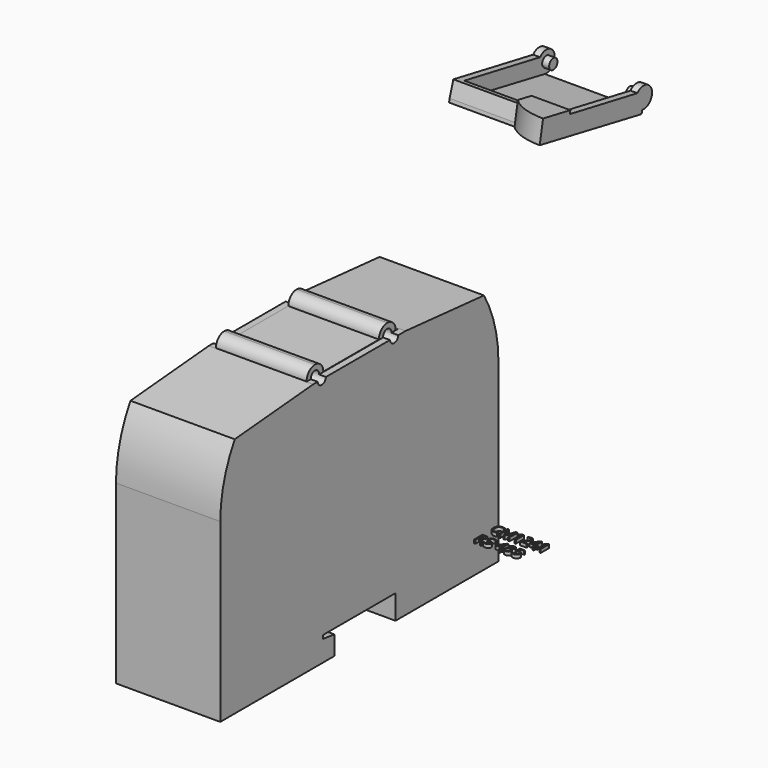
from build123d import *

# Parameters (mm, degrees)
F0_W          = 100
F0_H          = 75
F1_DEPTH      = 15
F3_DEPTH      = 34.2
F5_DEPTH      = 38.1
F6_W          = 4
F6_H          = 12
F7_DEPTH      = 10
F9_DEPTH      = 30
F10_W         = 26
F10_H         = 30.2941333291
F10_H_2       = 4.7058666709
F11_DEPTH     = 25
F12_R         = 1.5
F13_DEPTH     = 2
F14_R         = 1.5
F15_DEPTH     = 2
F16_W         = 26
F16_H         = 30.2941333291
F17_DEPTH     = 1
F19_DEPTH     = 6.4
F20_TEXT_SIZE = 4.1666666667
F21_DEPTH     = 1
F23_DEPTH     = 97.5
F25_DEPTH     = 45


# Not quite as in the source:
# - a feature names something its author has since deleted; it is built from what else it names
# - Text() gives the source's letters only with a copy of the font that has no kerning and outlines rounded to 1/6400 em; it was checked with that copy


with BuildPart() as f1:
    # F0 (on Right) → F1 (new body, symmetric)
    with BuildSketch(Plane.YZ):
        Rectangle(F0_W, F0_H)
    extrude(amount=F1_DEPTH, both=True)

    # F2 (on face) → F3 (cut)
    with BuildSketch(Plane.YZ.offset(15)):
        with BuildLine():
            ThreePointArc((-16.5, 34.5), (-15.62132033, 36.6213203571), (-13.4999999617, 37.5))
            Line((-13.4999999617, 37.5), (-50, 37.5))
            Line((-50, 37.5), (-50, 31.5))
            Line((-50, 31.5), (-16.4987426642, 34.4131528118))
            ThreePointArc((-16.4987426642, 34.4131528118), (-16.4996856496, 34.4565718554), (-16.5, 34.5))
        make_face()
        with BuildLine():
            ThreePointArc((12.5000000383, 37.5), (14.6213203571, 36.62132033), (15.5, 34.5))
            Line((15.5, 34.5), (50, 31.5))
            Line((50, 31.5), (50, 37.5))
            Line((50, 37.5), (12.5000000383, 37.5))
        make_face()
        with BuildLine():
            Line((-10.5, 34.5), (9.5, 34.5))
            ThreePointArc((9.5, 34.5), (10.37867967, 36.6213203571), (12.5000000383, 37.5))
            Line((12.5000000383, 37.5), (-13.4999999617, 37.5))
            ThreePointArc((-13.4999999617, 37.5), (-11.3786796429, 36.62132033), (-10.5, 34.5))
        make_face()
        with BuildLine():
            ThreePointArc((-15, 34.5), (-13.5, 33), (-12, 34.5))
            Line((-12, 34.5), (-15, 34.5))
        make_face()
        with BuildLine():
            Line((-15, 34.5), (-12, 34.5))
            ThreePointArc((-12, 34.5), (-13.5, 36), (-15, 34.5))
        make_face()
        with BuildLine():
            Line((14, 34.5), (11, 34.5))
            ThreePointArc((11, 34.5), (12.5, 33), (14, 34.5))
        make_face()
        with BuildLine():
            ThreePointArc((14, 34.5), (12.5, 36), (11, 34.5))
            Line((11, 34.5), (14, 34.5))
        make_face()
    extrude(amount=-F3_DEPTH, mode=Mode.SUBTRACT)

    # F4 (on face) → F5 (cut)
    with BuildSketch(Plane.YZ.offset(15)):
        with BuildLine():
            ThreePointArc((44.7955449747, 31.9525613065), (48.6477397083, 22.9432016728), (50, 13.2385967153))
            Line((50, 13.2385967153), (50, 31.5))
            Line((50, 31.5), (44.7955449747, 31.9525613065))
        make_face()
        with BuildLine():
            Line((-50, 31.5), (-50, 13.2385967153))
            ThreePointArc((-50, 13.2385967153), (-48.6477397083, 22.9432016728), (-44.7955449747, 31.9525613065))
            Line((-44.7955449747, 31.9525613065), (-50, 31.5))
        make_face()
    extrude(amount=-F5_DEPTH, mode=Mode.SUBTRACT)

    # F6 (on face) → F7 (cut)
    with BuildSketch(Plane(origin=(0, 50, 0), x_dir=(-1, 0, 0), z_dir=(0, 1, 0))):
        with Locations((-8, 2.2385967153)):
            Rectangle(F6_W, F6_H)
        with Locations((0, 2.2385967153)):
            Rectangle(F6_W, F6_H)
        with Locations((8, 2.2385967153)):
            Rectangle(F6_W, F6_H)
        with Locations((0, -17.7614032847)):
            Rectangle(F6_W, F6_H)
        with Locations((-8, -17.7614032847)):
            Rectangle(F6_W, F6_H)
        with Locations((8, -17.7614032847)):
            Rectangle(F6_W, F6_H)
    extrude(amount=-F7_DEPTH, mode=Mode.SUBTRACT)

    # F22 (on face) → F23 (cut)
    with BuildSketch(Plane.XZ.offset(50)):
        Polygon((-15.2735952288, 39.051361382), (-15.0366695598, 34.4017036259), (-13.0366695598, 34.4017036259), (-13.0366695598, 39.051361382), align=None)
        Polygon((13.0366695598, 39.051361382), (13.0366695598, 34.4017036259), (15.0366695598, 34.4017036259), (15.2735952288, 39.051361382), align=None)
    extrude(amount=-F23_DEPTH, mode=Mode.SUBTRACT)

    # F24 (on face) → F25 (cut)
    with BuildSketch(Plane(origin=(-15, 0, 0), x_dir=(0, -1, 0), z_dir=(-1, 0, 0))):
        Polygon((13, -30.5), (0, -30.5), (-13, -30.5), (-13, -37.5), (9, -37.5), (9, -32), (13, -31.5), align=None)
    extrude(amount=-F25_DEPTH, mode=Mode.SUBTRACT)


with BuildPart() as f9:
    # F8 (on Right) → F9 (new body)
    with BuildSketch(Plane.YZ):
        with BuildLine():
            Line((81.2311347941, 73.227164829), (52.5394231081, 78.6369070411))
            Line((52.5394231081, 78.6369070411), (51.1991754174, 74.3648558855))
            Line((51.1991754174, 74.3648558855), (82.9181422255, 68.2970562757))
            ThreePointArc((82.9181422255, 68.2970562757), (80.6433943819, 70.2723607925), (81.2311347941, 73.227164829))
        make_face()
        with BuildLine():
            ThreePointArc((86.4818173254, 71.2436255319), (84.5419947648, 74.0500509802), (81.2311347941, 73.227164829))
            ThreePointArc((81.2311347941, 73.227164829), (80.6433943819, 70.2723607925), (82.9181422255, 68.2970562757))
            ThreePointArc((82.9181422255, 68.2970562757), (85.3934886754, 68.9315890595), (86.4818173254, 71.2436255319))
        make_face()
    extrude(amount=F9_DEPTH)

    # F10 (on face) → F11 (cut)
    with BuildSketch(Plane(origin=(0, 15.5311841866, 81.1880990442), x_dir=(1, 0, 0), z_dir=(0, -0.1878917, -0.9821897521))):
        with Locations((15, -53.461832885)):
            Rectangle(F10_W, F10_H)
        with Locations((15, -70.961832885)):
            Rectangle(F10_W, F10_H_2)
    extrude(amount=-F11_DEPTH, mode=Mode.SUBTRACT)

    # F12 (on face) → F13 (join)
    with BuildSketch(Plane.YZ.offset(2)):
        with Locations((83.4818173254, 71.2436255319)):
            Circle(F12_R)
    extrude(amount=F13_DEPTH)

    # F14 (on face) → F15 (join)
    with BuildSketch(Plane(origin=(28, 0, 0), x_dir=(0, -1, 0), z_dir=(-1, 0, 0))):
        with Locations((-83.4818173254, 71.2436255319)):
            Circle(F14_R)
    extrude(amount=F15_DEPTH)

    # F16 (on face) → F17 (join)
    with BuildSketch(Plane(origin=(0, 15.5311841866, 81.1880990442), x_dir=(1, 0, 0), z_dir=(0, -0.1878917, -0.9821897521))):
        with Locations((15, -53.461832885)):
            Rectangle(F16_W, F16_H)
        Polygon((30, -68.6088995496), (30, -36.3147662204), (0, -36.3147662204), (0, -68.6088995496), (2, -68.6088995496), (2, -38.3147662204), (28, -38.3147662204), (28, -68.6088995496), align=None)
    extrude(amount=F17_DEPTH)

    # F18 (on face) → F19 (join)
    with BuildSketch(Plane(origin=(0, 15.3432924866, 80.2059092921), x_dir=(1, 0, 0), z_dir=(0, -0.1878917, -0.9821897521))):
        with BuildLine():
            ThreePointArc((30, -31.3147662204), (23.876275643, -32.6217022828), (18.8196601125, -36.3147662204))
            Line((18.8196601125, -36.3147662204), (30, -36.3147662204))
            Line((30, -36.3147662204), (30, -31.3147662204))
        make_face()
        with BuildLine():
            ThreePointArc((30, -36.3147662204), (25, -37.6545121826), (21.3397459622, -41.3147662204))
            Line((21.3397459622, -41.3147662204), (30, -41.3147662204))
            Line((30, -41.3147662204), (30, -36.3147662204))
        make_face()
        with BuildLine():
            Line((18.8196601125, -36.3147662204), (18.8196601125, -41.3147662204))
            Line((18.8196601125, -41.3147662204), (21.3397459622, -41.3147662204))
            ThreePointArc((21.3397459622, -41.3147662204), (25, -37.6545121826), (30, -36.3147662204))
            Line((30, -36.3147662204), (18.8196601125, -36.3147662204))
        make_face()
    extrude(amount=-F19_DEPTH)


with BuildPart() as f21:
    # F20 (on Top) → F21 (new body)
    with BuildSketch(Plane.XY):
        with Locations((49.8833220437, 2.8602550319)):
            Text('CM1241', F20_TEXT_SIZE, font='Open Sans', text_align=(TextAlign.LEFT, TextAlign.BOTTOM))
        with Locations((49.8833220437, -2.8064116347)):
            Text('RS 485', F20_TEXT_SIZE, font='Open Sans', text_align=(TextAlign.LEFT, TextAlign.BOTTOM))
    extrude(amount=F21_DEPTH)


solid = Compound([f1.part, f9.part, f21.part])
